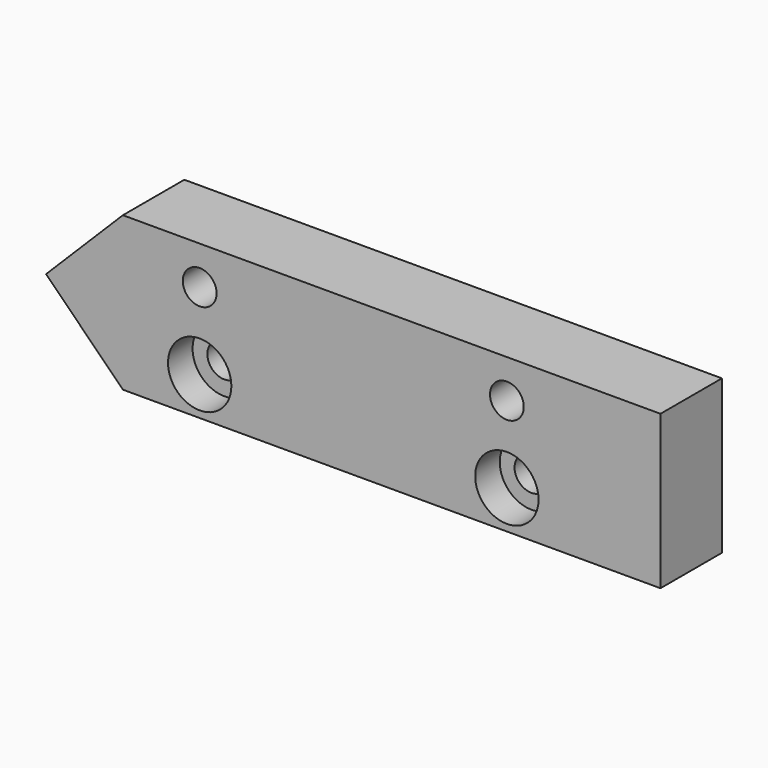
from build123d import *

# Parameters (mm, degrees)
F1_DEPTH       = 10
F3_D           = 4.4
F3_CBORE_D     = 8.25
F3_CBORE_DEPTH = 4
F5_D           = 4.4


# Not quite as in the source:
# - a feature names something its author has since deleted; it is built from what else it names


with BuildPart() as f1:
    # F0 (on Front) → F1 (new body)
    with BuildSketch(Plane.XZ):
        Polygon((-80, 10), (0, 10), (0, 20), (-70, 20), align=None)
        Polygon((-70, 0), (0, 0), (0, 10), (-80, 10), align=None)
    extrude(amount=F1_DEPTH)

    # F3 (through all)
    with Locations(Plane.XZ.offset(10)):
        with Locations((-20, 5), (-60, 5)):
            CounterBoreHole(F3_D / 2, F3_CBORE_D / 2, F3_CBORE_DEPTH)

    # F5 (through all)
    with Locations(Plane.XZ.offset(10)):
        with Locations((-60, 15), (-20, 15)):
            Hole(F5_D / 2)


solid = f1.part
